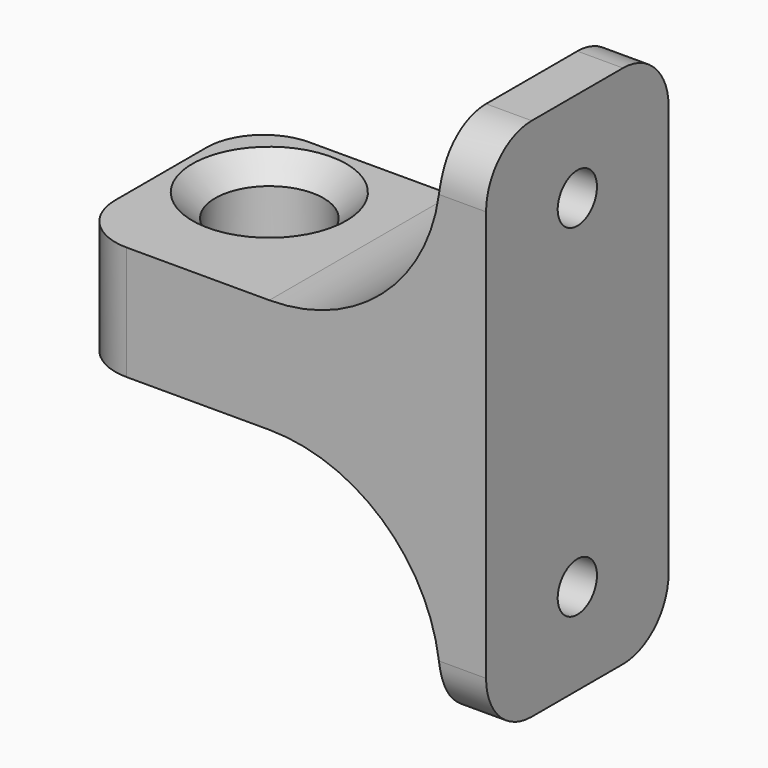
from build123d import *

# Parameters (mm, degrees)
F0_W          = 36.5
F0_H          = 20
F0_R          = 4.75
F1_DEPTH      = 5
F1_DEPTH_BACK = 5
F2_SIZE       = 2
F3_W          = 20
F3_H          = 46
F3_R          = 4
F4_DEPTH      = 4
F5_T4_DEPTH   = 20
F5_S5_R       = 4
F5_T6_DEPTH   = 16
F5_T10_DEPTH  = 20
F5_S11_R      = 4
F5_T12_DEPTH  = 16
F3_R_2        = 2.15
F6_DEPTH      = 4
F7_R          = 5
F8_R          = 5


# Not quite as in the source:
# - a fillet or chamfer that OpenCascade refuses, or shapes differently, is made with other operations: its cross-section is extruded or revolved along the edge and cut away or added


with BuildPart() as f1:
    # F0 (on Top) → F1 (new body, two sides)
    with BuildSketch(Plane.XY) as f1_sk:
        with Locations((-18.25, -2.5)):
            Rectangle(F0_W, F0_H)
        with Locations((-29, 0)):
            Circle(F0_R, mode=Mode.SUBTRACT)
    extrude(amount=F1_DEPTH)
    extrude(f1_sk.sketch, amount=-F1_DEPTH_BACK)

    # F2
    f2_edges = [f1.edges().sort_by_distance(p)[0] for p in [
        (-33.75, 0, 5),
        (-33.75, 0, -5),
    ]]
    chamfer(f2_edges, length=F2_SIZE)

    # F3 (on Right) → F4 (join)
    with BuildSketch(Plane.YZ):
        with Locations((-2.5, 0)):
            Rectangle(F3_W, F3_H)
        with Locations((-2.5, -15)):
            Circle(F3_R, mode=Mode.SUBTRACT)
        with Locations((-2.5, 15)):
            Circle(F3_R, mode=Mode.SUBTRACT)
    extrude(amount=-F4_DEPTH)

    # F5: fillet of radius 15 on 2 edges, made by hand


with BuildPart() as f5_tool2:
    # F5_s3 → F5_t4 (new body)
    with BuildSketch(Plane.XZ.offset(12.5)):
        with BuildLine():
            ThreePointArc((-19, 5), (-8.3933982822, 9.3933982822), (-4, 20))
            Line((-4, 20), (-4, 5))
            Line((-4, 5), (-19, 5))
        make_face()
    extrude(amount=-F5_T4_DEPTH)

    # F5_s5 → F5_t6 (cut, symmetric)
    with BuildSketch(Plane.YZ.offset(-11.5)):
        with Locations((-2.5, 15)):
            Circle(F5_S5_R)
    extrude(amount=F5_T6_DEPTH, both=True, mode=Mode.SUBTRACT)


with BuildPart() as f1_1:
    add(f1.part)

    # F5_t1: union F5_tool2
    add(f5_tool2.part)


with BuildPart() as f5_tool8:
    # F5_s9 → F5_t10 (new body)
    with BuildSketch(Plane.XZ.offset(12.5)):
        with BuildLine():
            ThreePointArc((-4, -20), (-8.3933982822, -9.3933982822), (-19, -5))
            Line((-19, -5), (-4, -5))
            Line((-4, -5), (-4, -20))
        make_face()
    extrude(amount=-F5_T10_DEPTH)

    # F5_s11 → F5_t12 (cut, symmetric)
    with BuildSketch(Plane.YZ.offset(-11.5)):
        with Locations((-2.5, -15)):
            Circle(F5_S11_R)
    extrude(amount=F5_T12_DEPTH, both=True, mode=Mode.SUBTRACT)


with BuildPart() as f1_2:
    add(f1_1.part)

    # F5_t7: union F5_tool8
    add(f5_tool8.part)

    # F3 (on Right) → F6 (join)
    with BuildSketch(Plane.YZ):
        with Locations((-2.5, 15)):
            Circle(F3_R)
        with Locations((-2.5, 15)):
            Circle(F3_R_2, mode=Mode.SUBTRACT)
        with Locations((-2.5, -15)):
            Circle(F3_R)
        with Locations((-2.5, -15)):
            Circle(F3_R_2, mode=Mode.SUBTRACT)
    extrude(amount=-F6_DEPTH)

    # F7
    f7_edges = [f1_2.edges().sort_by_distance(p)[0] for p in [
        (-2, -12.5, -23),
        (-2, -12.5, 23),
        (-2, 7.5, -23),
        (-2, 7.5, 23),
    ]]
    fillet(f7_edges, radius=F7_R)

    # F8
    f8_edges = [f1_2.edges().sort_by_distance(p)[0] for p in [
        (-36.5, -12.5, 0),
        (-36.5, 7.5, 0),
    ]]
    fillet(f8_edges, radius=F8_R)


solid = f1_2.part
